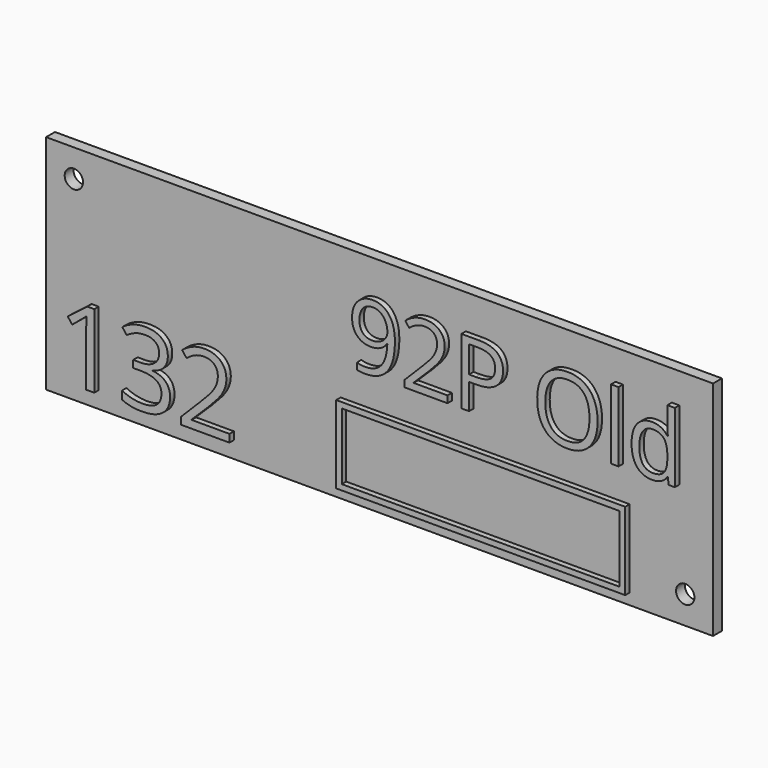
from build123d import *

# Parameters (mm, degrees)
F0_W         = 120
F0_H         = 40
F1_DEPTH     = 2
F3_D         = 3.3
F4_TEXT_SIZE = 16.5346193593
F5_DEPTH     = 1
F6_TEXT_SIZE = 18.5356140827
F7_DEPTH     = 1
F8_W         = 52
F8_H         = 14
F8_W_2       = 49.99999962
F8_H_2       = 11.99999962
F9_DEPTH     = 1


# Not quite as in the source:
# - Text() gives the source's letters only with a copy of the font that has no kerning and outlines rounded to 1/6400 em; it was checked with that copy


with BuildPart() as f1:
    # F0 (on Front) → F1 (new body)
    with BuildSketch(Plane.XZ):
        Rectangle(F0_W, F0_H)
    extrude(amount=F1_DEPTH)

    # F3 (through all)
    with Locations(Plane.XZ.offset(2)):
        with Locations((-55, 15), (55, -15)):
            Hole(F3_D / 2)

    # F4 (on face) → F5 (join)
    with BuildSketch(Plane.XZ.offset(2)):
        with Locations((-5, 2)):
            Text('92P Old', F4_TEXT_SIZE, font='Open Sans', text_align=(TextAlign.LEFT, TextAlign.BOTTOM))
    extrude(amount=F5_DEPTH)

    # F6 (on face) → F7 (join)
    with BuildSketch(Plane.XZ.offset(2)):
        with Locations((-57, -17)):
            Text('132', F6_TEXT_SIZE, font='Open Sans', text_align=(TextAlign.LEFT, TextAlign.BOTTOM))
    extrude(amount=F7_DEPTH)

    # F8 (on face) → F9 (join)
    with BuildSketch(Plane.XZ.offset(2)):
        with Locations((19, -11)):
            Rectangle(F8_W, F8_H)
        with Locations((19, -11)):
            Rectangle(F8_W_2, F8_H_2, mode=Mode.SUBTRACT)
    extrude(amount=F9_DEPTH)


solid = f1.part
